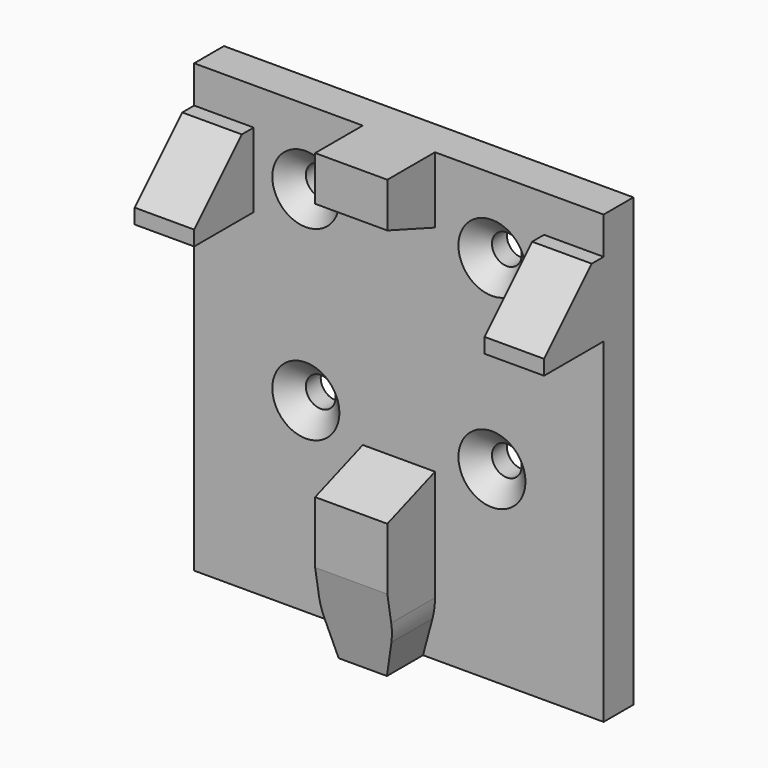
from build123d import *

# Parameters (mm, degrees)
F1_DEPTH       = 60
F3_D           = 4
F3_CSINK_D     = 9
F3_CSINK_ANGLE = 90
F4_C1_SIZE2    = 1.6076951546
F4_C1_SIZE     = 6
F4_C2_SIZE2    = 6
F4_C2_SIZE     = 1.6076951546
F6_R           = 10
F5_W           = 8
F5_H           = 10
F7_DEPTH       = 10
F8_SIZE        = 8
F10_DEPTH      = 9.7
F11_SIZE2      = 1.9395967878
F11_SIZE       = 11


# Not quite as in the source:
# - a feature names something its author has since deleted; it is built from what else it names


with BuildPart() as f1:
    # F0 (on Top) → F1 (new body)
    with BuildSketch(Plane.XY):
        Polygon((4.85, 0), (27.5, 0), (27.5, 5), (-27.5, 5), (-27.5, 0), (-4.85, 0), (-4.85, -8), (4.85, -8), align=None)
    extrude(amount=F1_DEPTH)

    # F3 (through all)
    with Locations(Plane.XZ):
        with Locations((-12.5, 50), (-12.5, 25), (12.5, 50), (12.5, 25)):
            CounterSinkHole(F3_D / 2, F3_CSINK_D / 2, counter_sink_angle=F3_CSINK_ANGLE)

    # F4: chamfer of 6 x 1.6076951546 on 2 edges, made by hand

    # F4_c1
    f4_c1_edges = [f1.edges().sort_by_distance(p)[0] for p in [
        (4.85, -4, 0),
    ]]
    f4_c1_side = f1.faces().sort_by_distance((4.85, -4, 0.0321539031))[0]
    chamfer(f4_c1_edges, length=F4_C1_SIZE, length2=F4_C1_SIZE2, reference=f4_c1_side)

    # F4_c2
    f4_c2_edges = [f1.edges().sort_by_distance(p)[0] for p in [
        (-4.85, -4, 0),
    ]]
    f4_c2_side = f1.faces().sort_by_distance((-4.8178460969, -4, 0))[0]
    chamfer(f4_c2_edges, length=F4_C2_SIZE, length2=F4_C2_SIZE2, reference=f4_c2_side)

    # F6
    f6_edges = [f1.edges().sort_by_distance(p)[0] for p in [
        (-4.85, -4, 6),
        (4.85, -4, 6),
    ]]
    fillet(f6_edges, radius=F6_R)

    # F5 (on face) → F7 (join)
    with BuildSketch(Plane.XZ):
        with Locations((-23.5, 50)):
            Rectangle(F5_W, F5_H)
        with Locations((23.5, 50)):
            Rectangle(F5_W, F5_H)
    extrude(amount=F7_DEPTH)

    # F8
    f8_edges = [f1.edges().sort_by_distance(p)[0] for p in [
        (-23.5, -10, 55),
        (23.5, -10, 55),
    ]]
    chamfer(f8_edges, length=F8_SIZE)

    # F9 (on face) → F10 (cut, through all)
    with BuildSketch(Plane.YZ.offset(4.85)):
        Polygon((0, 51.0882381259), (-8, 54), (-8, 19.3165249759), (0, 22.22828685), align=None)
    extrude(amount=-F10_DEPTH, mode=Mode.SUBTRACT)

    # F11
    f11_edges = [f1.edges().sort_by_distance(p)[0] for p in [
        (0, -8, 0),
    ]]
    f11_side = f1.faces().sort_by_distance((0, -8, 10.07737))[0]
    chamfer(f11_edges, length=F11_SIZE, length2=F11_SIZE2, reference=f11_side)


solid = f1.part
